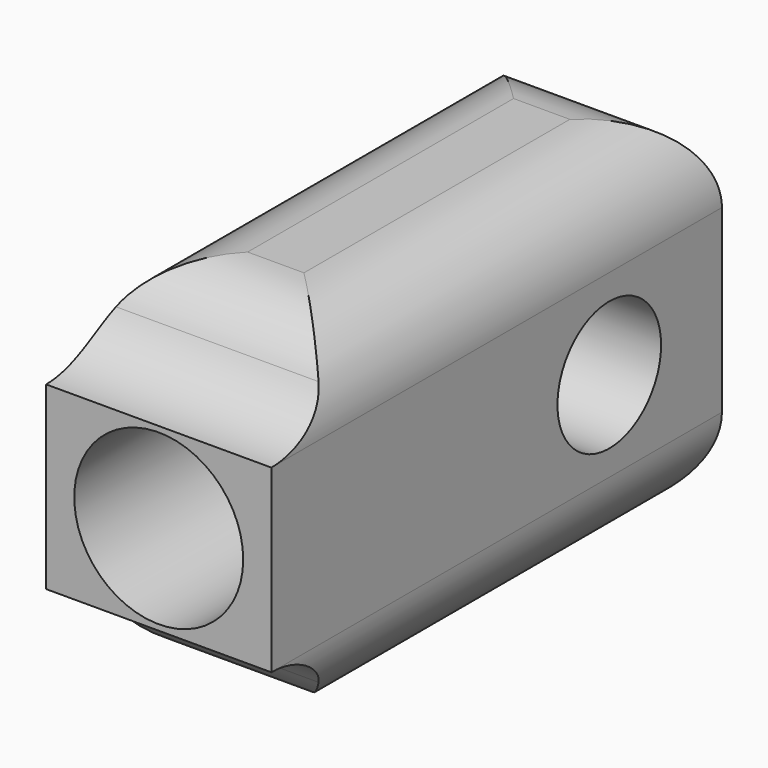
from build123d import *

# Parameters (mm, degrees)
F0_R     = 1.15
F1_DEPTH = 2
F2_R     = 1.5
F3_DEPTH = 5
F4_R     = 1.49999


# Not quite as in the source:
# - a fillet or chamfer is up to 0.001 mm smaller than in the source, because OpenCascade refuses the exact size


with BuildPart() as f1:
    # F0 (on Right) → F1 (new body, symmetric)
    with BuildSketch(Plane.YZ):
        with BuildLine():
            Line((5, -3.1), (5, 3.1))
            Line((5, 3.1), (-3.5, 3.1))
            ThreePointArc((-3.5, 3.1), (-3.9393398282, 2.0393398282), (-5, 1.6))
            Line((-5, 1.6), (-5, -1.6))
            ThreePointArc((-5, -1.6), (-3.9393398282, -2.0393398282), (-3.5, -3.1))
            Line((-3.5, -3.1), (5, -3.1))
        make_face()
        with Locations((2.5, 0)):
            Circle(F0_R, mode=Mode.SUBTRACT)
    extrude(amount=F1_DEPTH, both=True)

    # F2 (on face) → F3 (cut)
    with BuildSketch(Plane.XZ.offset(5)):
        Circle(F2_R)
    extrude(amount=-F3_DEPTH, mode=Mode.SUBTRACT)

    # F4 (radius 1.5 in the source; OpenCascade refuses exactly that, so slightly less here)
    f4_edges = [f1.edges().sort_by_distance(p)[0] for p in [
        (0, -3.5, 3.1),
        (0, -3.5, -3.1),
        (2, 0.75, -3.1),
        (2, 0.75, 3.1),
        (0, 5, 3.1),
        (0, 5, -3.1),
        (-2, 0.75, 3.1),
        (-2, 0.75, -3.1),
    ]]
    fillet(f4_edges, radius=F4_R)


solid = f1.part
